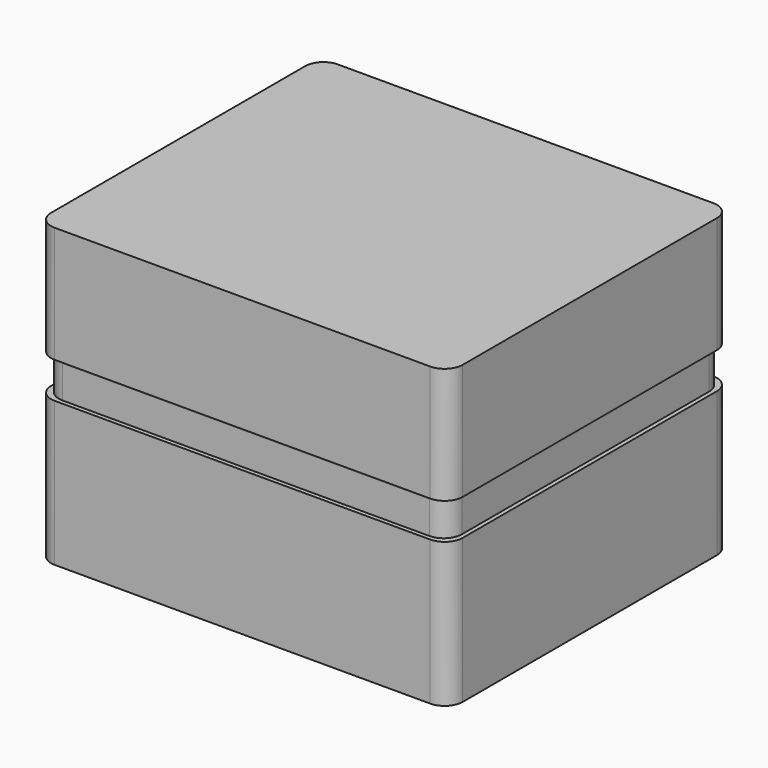
from build123d import *

# Parameters (mm, degrees)
F0_W          = 114
F0_H          = 98
F0_W_2        = 13
F0_H_2        = 37
F0_W_3        = 17.5
F0_H_3        = 13
F0_W_4        = 22
F0_H_4        = 8
F1_DEPTH      = 45
F2_W          = 114
F2_H          = 5
F3_DEPTH      = 98
F4_R          = 2
F19_DEPTH     = 8
F20_DEPTH     = 13
F21_DEPTH     = 37
F22_W         = 114
F22_H         = 98
F22_W_2       = 111.6
F22_H_2       = 95.6
F23_DEPTH     = 10
F24_R         = 1
F25_T1_DEPTH  = 65
F25_T3_DEPTH  = 10
F25_T6_ANGLE  = 90
F25_T8_ANGLE  = 90
F25_T10_ANGLE = 90
F25_T12_ANGLE = 90
F26_DEPTH     = 9.2
F27_W         = 114
F27_H         = 98
F27_W_2       = 111.6
F27_H_2       = 95.6
F27_W_3       = 108
F27_H_3       = 92
F28_DEPTH     = 20
F29_W         = 114
F29_H         = 3
F30_DEPTH     = 98
F31_R         = 5


# Not quite as in the source:
# - a fillet or chamfer that OpenCascade refuses, or shapes differently, is made with other operations: its cross-section is extruded or revolved along the edge and cut away or added


with BuildPart() as f1:
    # F0 (on Top) → F1 (new body)
    with BuildSketch(Plane.XY):
        with Locations((-13.5, 0)):
            Rectangle(F0_W, F0_H)
        with Locations((-55.5, -19.9149964719)):
            Rectangle(F0_W_2, F0_H_2, mode=Mode.SUBTRACT)
        Polygon((34.5, -35), (34.5, -45), (31.5, -45), (31.5, -35), (26.5, -35), (26.5, -45), (23.5, -45), (23.5, -35), (18.5, -35), (18.5, -45), (15.5, -45), (15.5, -35), (10.5, -35), (10.5, -45), (7.5, -45), (7.5, -35), (2.5, -35), (2.5, -45), (0.5, -45), (0.5, -35), (-4.5, -35), (-4.5, -45), (-34.5, -45), (-34.5, -35), (-39.5, -35), (-39.5, 35), (-34.5, 35), (-34.5, 45), (-4.5, 45), (-4.5, 35), (0.5, 35), (0.5, 45), (2.5, 45), (2.5, 35), (7.5, 35), (7.5, 45), (10.5, 45), (10.5, 35), (15.5, 35), (15.5, 45), (18.5, 45), (18.5, 35), (23.5, 35), (23.5, 45), (26.5, 45), (26.5, 35), (31.5, 35), (31.5, 45), (34.5, 45), (34.5, 35), (39.5, 35), (39.5, -35), align=None, mode=Mode.SUBTRACT)
        with Locations((-55.5, 15.0850035281)):
            Rectangle(F0_W_3, F0_H_3, mode=Mode.SUBTRACT)
        with Locations((-55.5, 35.5850035281)):
            Rectangle(F0_W_4, F0_H_4, mode=Mode.SUBTRACT)
        with Locations((-55.5, 35.5850035281)):
            Rectangle(F0_W_4, F0_H_4)
        with Locations((-55.5, 15.0850035281)):
            Rectangle(F0_W_3, F0_H_3)
        with Locations((-55.5, -19.9149964719)):
            Rectangle(F0_W_2, F0_H_2)
    extrude(amount=-F1_DEPTH)

    # F2 (on face) → F3 (join, through all)
    with BuildSketch(Plane.XZ.offset(49)):
        with Locations((-13.5, -47.5)):
            Rectangle(F2_W, F2_H)
    extrude(amount=-F3_DEPTH)

    # F4
    f4_edges = [f1.edges().sort_by_distance(p)[0] for p in [
        (-34.5, 35, -22.5),
        (-4.5, 35, -22.5),
        (0.5, 35, -22.5),
        (2.5, 35, -22.5),
        (7.5, 35, -22.5),
        (10.5, 35, -22.5),
        (15.5, 35, -22.5),
        (18.5, 35, -22.5),
        (23.5, 35, -22.5),
        (26.5, 35, -22.5),
        (31.5, 35, -22.5),
        (34.5, 35, -22.5),
        (-34.5, -35, -22.5),
        (-4.5, -35, -22.5),
        (0.5, -35, -22.5),
        (2.5, -35, -22.5),
        (7.5, -35, -22.5),
        (10.5, -35, -22.5),
        (15.5, -35, -22.5),
        (18.5, -35, -22.5),
        (23.5, -35, -22.5),
        (26.5, -35, -22.5),
        (31.5, -35, -22.5),
        (34.5, -35, -22.5),
    ]]
    fillet(f4_edges, radius=F4_R)

    # F12 (on plane+point) → F19 (cut, through all)
    with BuildSketch(Plane.XZ.offset(-31.5850035281)):
        Polygon((-44.5, -6.3508529611), (-44.5, 6.3508529611), (-55.5, 12.7017059222), (-66.5, 6.3508529611), (-66.5, -6.3508529611), (-55.5, -12.7017059222), align=None)
    extrude(amount=-F19_DEPTH, mode=Mode.SUBTRACT)

    # F15 (on plane+point) → F20 (cut, through all)
    with BuildSketch(Plane.XZ.offset(-8.5850035281)):
        Polygon((-46.75, -5.0518148554), (-46.75, 5.0518148554), (-55.5, 10.1036297108), (-64.25, 5.0518148554), (-64.25, -5.0518148554), (-55.5, -10.1036297108), align=None)
    extrude(amount=-F20_DEPTH, mode=Mode.SUBTRACT)

    # F18 (on plane+point) → F21 (cut, through all)
    with BuildSketch(Plane.XZ.offset(38.4149964719)):
        Polygon((-49, -3.7527767497), (-49, 3.7527767497), (-55.5, 7.5055534995), (-62, 3.7527767497), (-62, -3.7527767497), (-55.5, -7.5055534995), align=None)
    extrude(amount=-F21_DEPTH, mode=Mode.SUBTRACT)

    # F22 (on face) → F23 (cut)
    with BuildSketch(Plane.XY):
        with Locations((-13.5, 0)):
            Rectangle(F22_W, F22_H)
        with Locations((-13.5, 0)):
            Rectangle(F22_W_2, F22_H_2, mode=Mode.SUBTRACT)
    extrude(amount=-F23_DEPTH, mode=Mode.SUBTRACT)

    # F24
    f24_edges = [f1.edges().sort_by_distance(p)[0] for p in [
        (-69.3, 0, 0),
        (-13.5, 47.8, 0),
        (42.3, 0, 0),
        (-13.5, -47.8, 0),
        (-49, -19.914996, 0),
        (-55.5, -38.414996, 0),
        (-55.5, -1.414996, 0),
        (-62, -19.914996, 0),
        (-46.75, 15.085004, 0),
        (-55.5, 8.585004, 0),
        (-55.5, 21.585004, 0),
        (-64.25, 15.085004, 0),
        (-44.5, 35.585004, 0),
        (-55.5, 31.585004, 0),
        (-55.5, 39.585004, 0),
        (-66.5, 35.585004, 0),
        (34.5, -41, 0),
        (35.085786, -35.585786, 0),
        (33, -45, 0),
        (38, -35, 0),
        (31.5, -41, 0),
        (39.5, 0, 0),
        (30.914214, -35.585786, 0),
        (38, 35, 0),
        (29, -35, 0),
        (35.085786, 35.585786, 0),
        (27.085786, -35.585786, 0),
        (34.5, 41, 0),
        (26.5, -41, 0),
        (33, 45, 0),
        (25, -45, 0),
        (31.5, 41, 0),
        (23.5, -41, 0),
        (30.914214, 35.585786, 0),
        (22.914214, -35.585786, 0),
        (29, 35, 0),
        (21, -35, 0),
        (27.085786, 35.585786, 0),
        (19.085786, -35.585786, 0),
        (26.5, 41, 0),
        (18.5, -41, 0),
        (25, 45, 0),
        (17, -45, 0),
        (23.5, 41, 0),
        (15.5, -41, 0),
        (22.914214, 35.585786, 0),
        (14.914214, -35.585786, 0),
        (21, 35, 0),
        (13, -35, 0),
        (19.085786, 35.585786, 0),
        (11.085786, -35.585786, 0),
        (18.5, 41, 0),
        (10.5, -41, 0),
        (17, 45, 0),
        (9, -45, 0),
        (15.5, 41, 0),
        (7.5, -41, 0),
        (14.914214, 35.585786, 0),
        (6.914214, -35.585786, 0),
        (13, 35, 0),
        (5, -35, 0),
        (11.085786, 35.585786, 0),
        (3.085786, -35.585786, 0),
        (10.5, 41, 0),
        (2.5, -41, 0),
        (9, 45, 0),
        (1.5, -45, 0),
        (7.5, 41, 0),
        (0.5, -41, 0),
        (6.914214, 35.585786, 0),
        (-0.085786, -35.585786, 0),
        (5, 35, 0),
        (-2, -35, 0),
        (3.085786, 35.585786, 0),
        (-3.914214, -35.585786, 0),
        (2.5, 41, 0),
        (-4.5, -41, 0),
        (1.5, 45, 0),
        (-19.5, -45, 0),
        (0.5, 41, 0),
        (-34.5, -41, 0),
        (-0.085786, 35.585786, 0),
        (-35.085786, -35.585786, 0),
        (-2, 35, 0),
        (-38, -35, 0),
        (-3.914214, 35.585786, 0),
        (-39.5, 0, 0),
        (-4.5, 41, 0),
        (-38, 35, 0),
        (-19.5, 45, 0),
        (-35.085786, 35.585786, 0),
        (-34.5, 41, 0),
    ]]
    fillet(f24_edges, radius=F24_R)

    # F25: fillet of radius 5 on 8 edges, made by hand

    # F25_s2 → F25_t1 (cut)
    with BuildSketch(Plane.XY.offset(-62.5)):
        with BuildLine():
            ThreePointArc((-70.5, -44), (-69.0355339059, -47.5355339059), (-65.5, -49))
            Line((-65.5, -49), (-70.5, -49))
            Line((-70.5, -49), (-70.5, -44))
        make_face()
        with BuildLine():
            ThreePointArc((-65.5, 49), (-69.0355339059, 47.5355339059), (-70.5, 44))
            Line((-70.5, 44), (-70.5, 49))
            Line((-70.5, 49), (-65.5, 49))
        make_face()
        with BuildLine():
            ThreePointArc((43.5, -44), (42.0355339059, -47.5355339059), (38.5, -49))
            Line((38.5, -49), (43.5, -49))
            Line((43.5, -49), (43.5, -44))
        make_face()
        with BuildLine():
            ThreePointArc((43.5, 44), (42.0355339059, 47.5355339059), (38.5, 49))
            Line((38.5, 49), (43.5, 49))
            Line((43.5, 49), (43.5, 44))
        make_face()
    extrude(amount=F25_T1_DEPTH, mode=Mode.SUBTRACT)

    # F25_s4 → F25_t3 (cut)
    with BuildSketch(Plane.XY.offset(-10)):
        with BuildLine():
            ThreePointArc((-69.3, -42.8), (-67.8355339059, -46.3355339059), (-64.3, -47.8))
            Line((-64.3, -47.8), (-69.3, -47.8))
            Line((-69.3, -47.8), (-69.3, -42.8))
        make_face()
        with BuildLine():
            ThreePointArc((-69.3, 42.8), (-67.8355339059, 46.3355339059), (-64.3, 47.8))
            Line((-64.3, 47.8), (-69.3, 47.8))
            Line((-69.3, 47.8), (-69.3, 42.8))
        make_face()
        with BuildLine():
            ThreePointArc((37.3, -47.8), (40.8355339059, -46.3355339059), (42.3, -42.8))
            Line((42.3, -42.8), (42.3, -47.8))
            Line((42.3, -47.8), (37.3, -47.8))
        make_face()
        with BuildLine():
            ThreePointArc((37.3, 47.8), (40.8355339059, 46.3355339059), (42.3, 42.8))
            Line((42.3, 42.8), (42.3, 47.8))
            Line((42.3, 47.8), (37.3, 47.8))
        make_face()
    extrude(amount=F25_T3_DEPTH, mode=Mode.SUBTRACT)

    # F25_s5 → F25_t6 (revolve, cut)
    with BuildSketch(Plane.XZ.offset(-42.8)):
        with BuildLine():
            ThreePointArc((41.3, 0), (42.0071067812, -0.2928932188), (42.3, -1))
            Line((42.3, -1), (42.3, 0))
            Line((42.3, 0), (41.3, 0))
        make_face()
    revolve(axis=Axis((37.3, 42.8, 0), (0, 0, 1)), revolution_arc=F25_T6_ANGLE, mode=Mode.SUBTRACT)

    # F25_s7 → F25_t8 (revolve, cut)
    with BuildSketch(Plane.YZ.offset(37.3)):
        with BuildLine():
            ThreePointArc((-46.8, 0), (-47.5071067812, -0.2928932188), (-47.8, -1))
            Line((-47.8, -1), (-47.8, 0))
            Line((-47.8, 0), (-46.8, 0))
        make_face()
    revolve(axis=Axis((37.3, -42.8, 0), (0, 0, 1)), revolution_arc=F25_T8_ANGLE, mode=Mode.SUBTRACT)

    # F25_s9 → F25_t10 (revolve, cut)
    with BuildSketch(Plane.YZ.offset(-64.3)):
        with BuildLine():
            ThreePointArc((46.8, 0), (47.5071067812, -0.2928932188), (47.8, -1))
            Line((47.8, -1), (47.8, 0))
            Line((47.8, 0), (46.8, 0))
        make_face()
    revolve(axis=Axis((-64.3, 42.8, 0), (0, 0, 1)), revolution_arc=F25_T10_ANGLE, mode=Mode.SUBTRACT)

    # F25_s11 → F25_t12 (revolve, cut)
    with BuildSketch(Plane.XZ.offset(42.8)):
        with BuildLine():
            ThreePointArc((-68.3, 0), (-69.0071067812, -0.2928932188), (-69.3, -1))
            Line((-69.3, -1), (-69.3, 0))
            Line((-69.3, 0), (-68.3, 0))
        make_face()
    revolve(axis=Axis((-64.3, -42.8, 0), (0, 0, 1)), revolution_arc=F25_T12_ANGLE, mode=Mode.SUBTRACT)


with BuildPart() as f26:
    # F22 (on face) → F26 (new body)
    with BuildSketch(Plane.XY):
        with Locations((-13.5, 0)):
            Rectangle(F22_W, F22_H)
        with Locations((-13.5, 0)):
            Rectangle(F22_W_2, F22_H_2, mode=Mode.SUBTRACT)
    extrude(amount=F26_DEPTH)

    # F27 (on face) → F28 (join)
    with BuildSketch(Plane.XY.offset(9.2)):
        with Locations((-13.5, 0)):
            Rectangle(F27_W, F27_H)
        with Locations((-13.5, 0)):
            Rectangle(F27_W_2, F27_H_2, mode=Mode.SUBTRACT)
        with Locations((-13.5, 0)):
            Rectangle(F27_W_2, F27_H_2)
        with Locations((-13.5, 0)):
            Rectangle(F27_W_3, F27_H_3, mode=Mode.SUBTRACT)
    extrude(amount=F28_DEPTH)

    # F29 (on face) → F30 (join, through all)
    with BuildSketch(Plane(origin=(0, 49, 0), x_dir=(-1, 0, 0), z_dir=(0, 1, 0))):
        with Locations((13.5, 30.7)):
            Rectangle(F29_W, F29_H)
    extrude(amount=-F30_DEPTH)

    # F31
    f31_edges = [f26.edges().sort_by_distance(p)[0] for p in [
        (43.5, -49, 16.1),
        (42.3, -47.8, 4.6),
        (40.5, 46, 19.2),
        (42.3, 47.8, 4.6),
        (-67.5, 46, 19.2),
        (-69.3, 47.8, 4.6),
        (-67.5, -46, 19.2),
        (-69.3, -47.8, 4.6),
        (-70.5, -49, 16.1),
        (-70.5, 49, 16.1),
        (43.5, 49, 16.1),
    ]]
    fillet(f31_edges, radius=F31_R)


solid = Compound([f1.part, f26.part])
